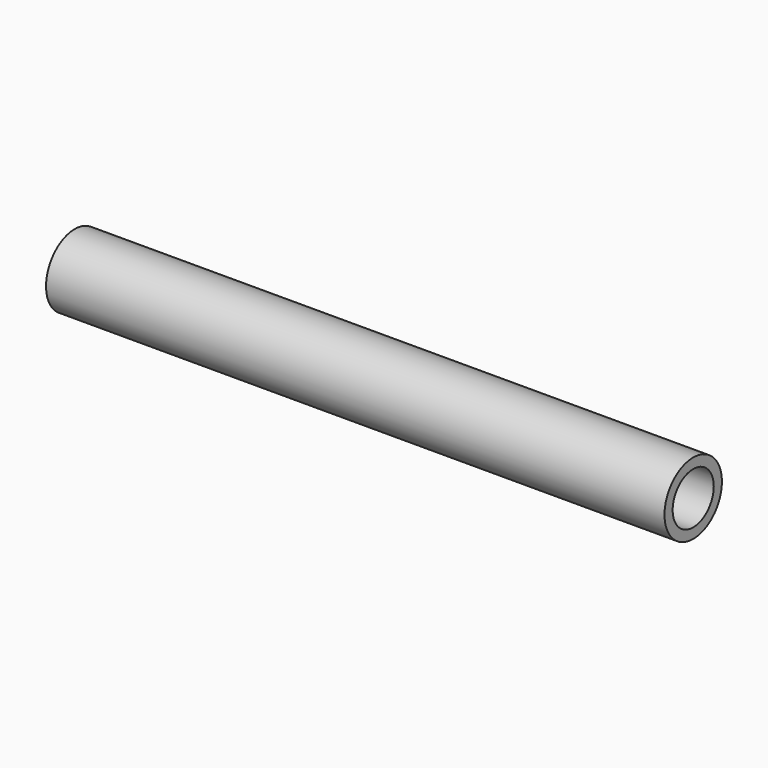
from build123d import *

# Parameters (mm, degrees)
F0_R     = 10.6426
F0_R_2   = 7.62
F1_DEPTH = 91.67749


# Not quite as in the source:
# - a length typed as a fraction of an inch, garbled in the dataset ("3 / 203.2 mm" for 3/8 in), is restored


with BuildPart() as f1:
    # F0 (on Right) → F1 (new body, symmetric)
    with BuildSketch(Plane.YZ):
        Circle(F0_R)
        Circle(F0_R_2, mode=Mode.SUBTRACT)
    extrude(amount=F1_DEPTH, both=True)


solid = f1.part
